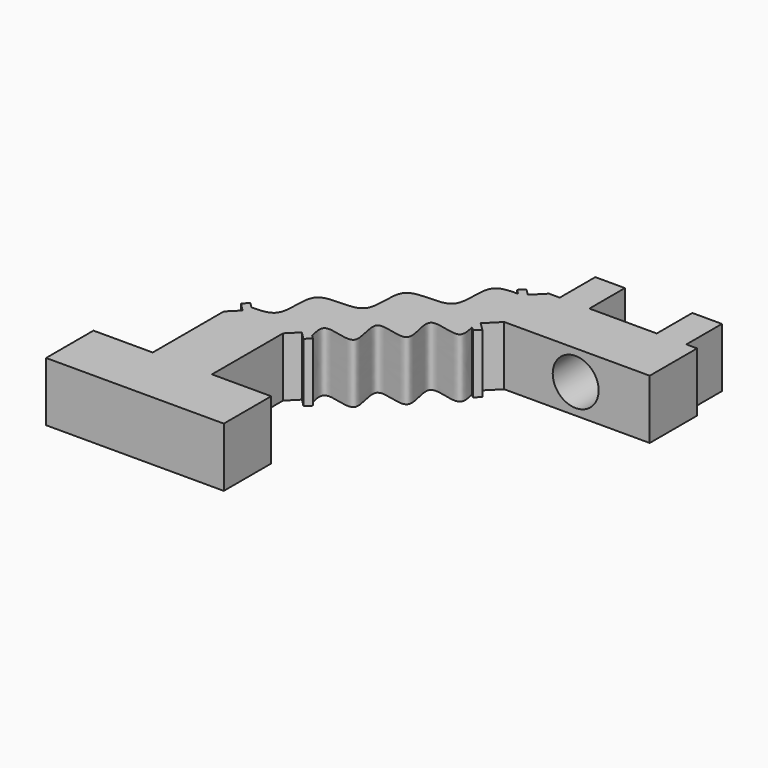
from build123d import *

# Parameters (mm, degrees)
F1_DEPTH = 4
F2_W     = 2
F2_H     = 4
F3_DEPTH = 3
F4_R     = 1.55
F5_DEPTH = 4


# Not quite as in the source:
# - ends of sketch curves that miss each other by under 0.0002 mm in the source are joined


with BuildPart() as f1:
    # F0 (on Top) → F1 (new body)
    with BuildSketch(Plane.XY):
        with BuildLine():
            Line((4, 0), (8, 0))
            Line((8, 0), (12, 0))
            Line((12, 0), (12, 4))
            Line((12, 4), (8, 4))
            Line((8, 4), (8, 10))
            Line((8, 10), (8.7071067812, 10.7071067812))
            Line((8.7071067812, 10.7071067812), (8.1767766953, 11.2374368671))
            Line((8.1767766953, 11.2374368671), (8.5303300859, 11.5909902577))
            Line((8.5303300859, 11.5909902577), (8.7778174593, 11.3435028843))
            add(Edge.make_bspline(
                [(8.7778174593, 11.3435028843), (8.6793135956, 11.7753291065), (8.4823058683, 12.638981551), (9.7777845344, 12.3434699588), (10.6414369797, 12.1464622341), (10.8080981583, 12.3131234115)],
                knots=[0, 0, 0, 0, 0.0833326877, 0.1666653755, 0.2499980632, 0.2499980632, 0.2499980632, 0.2499980632], degree=3))
            add(Edge.make_bspline(
                [(10.8080981583, 12.3131234115), (10.9747593369, 12.4797845889), (10.7777516061, 13.3434370232), (10.4822400343, 14.6389157463), (11.7777186285, 14.343403944), (13.0731975651, 14.047893141), (12.7776849661, 15.3433688663), (12.4821771366, 16.6388585097), (13.7776618368, 16.3433013729), (15.073233045, 16.047933522), (14.8762893212, 16.9116464302), (14.7778174593, 17.3435028843)],
                knots=[0.2499980632, 0.2499980632, 0.2499980632, 0.2499980632, 0.333330751, 0.4166634387, 0.4999961264, 0.5833288142, 0.6666615019, 0.7499941897, 0.8333268774, 0.9166634387, 1, 1, 1, 1], degree=3))
            Line((14.7778174593, 17.3435028843), (14.5303300859, 17.5909902577))
            Line((14.5303300859, 17.5909902577), (14.8838834765, 17.9445436483))
            Line((14.8838834765, 17.9445436483), (15.4142135624, 17.4142135624))
            Line((15.4142135624, 17.4142135624), (16.2980970389, 18.2980970389))
            Line((16.2980970389, 18.2980970389), (26.1212241882, 18.2980970389))
            Line((26.1212241882, 18.2980970389), (26.1212241882, 22.2980970389))
            Line((26.1212241882, 22.2980970389), (16.1212241882, 22.2980970389))
            Line((16.1212241882, 22.2980970389), (15.3256809034, 21.5025539105))
            Line((15.3256809034, 21.5025539105), (15.7675746595, 21.0606601544))
            Line((15.7675746595, 21.0606601544), (15.4140212689, 20.7071067638))
            Line((15.4140212689, 20.7071067638), (15.3257290593, 20.7953989734))
            Line((15.3257290593, 20.7953989734), (15.2726959638, 20.8484320689))
            add(Edge.make_bspline(
                [(5.2727919408, 10.8485280459), (5.8157320976, 10.8611381168), (6.9016124112, 10.8863582587), (6.939442624, 12.5151787291), (6.9772728368, 14.1439991996), (8.6060933073, 14.1818294124), (10.2349137777, 14.2196596252), (10.2727439905, 15.8484800956), (10.3105742033, 17.4773005661), (11.9393946738, 17.5151307789), (13.5682151443, 17.5529609917), (13.6060453571, 19.1817814621), (13.6438755698, 20.8106019326), (14.7297558835, 20.8358220745), (15.2726959638, 20.8484320689)],
                knots=[0, 0, 0, 0, 0.0833333333, 0.1666666667, 0.25, 0.3333333333, 0.4166666667, 0.5, 0.5833333333, 0.6666666667, 0.75, 0.8333333333, 0.9166666667, 1, 1, 1, 1], degree=3))
            Line((5.2727919408, 10.8485280459), (5.6282136765, 10.4931061393))
            Line((5.6282136765, 10.4931061393), (5.2746603207, 10.1395527139))
            Line((5.2746603207, 10.1395527139), (4.7071065842, 10.7071067232))
            Line((4.7071065842, 10.7071067232), (4, 10))
            Line((4, 10), (4, 4))
            Line((4, 4), (0, 4))
            Line((0, 4), (0, 0))
            Line((0, 0), (4, 0))
        make_face()
        Polygon((8.1767766953, 11.2374368671), (8.7071067812, 10.7071067812), (9.2374368671, 10.1767766953), (9.5909902577, 10.5303300859), (9.3435028843, 10.7778174593), (9.0606601718, 11.0606601718), (8.7778174593, 11.3435028843), (8.5303300859, 11.5909902577), align=None)
        Polygon((4.1395527627, 11.2746608175), (4.7071065842, 10.7071067232), (4.8838832621, 10.8838834359), (5.0606599574, 11.0606601312), (4.848527974, 11.2727922166), (4.7954948913, 11.3258253248), (4.4931062383, 11.6282141232), align=None)
        Polygon((4.8838832621, 10.8838834359), (4.7071065842, 10.7071067232), (5.2746603207, 10.1395527139), (5.6282136765, 10.4931061393), (5.2727919408, 10.8485280459), (5.0606599574, 11.0606601312), align=None)
        with BuildLine():
            Line((4.848527974, 11.2727922166), (5.0606599574, 11.0606601312))
            Line((5.0606599574, 11.0606601312), (5.2727919408, 10.8485280459))
            add(Edge.make_bspline(
                [(5.2727919408, 10.8485280459), (5.8157320976, 10.8611381168), (6.9016124112, 10.8863582587), (6.939442624, 12.5151787291), (6.9772728368, 14.1439991996), (8.6060933073, 14.1818294124), (10.2349137777, 14.2196596252), (10.2727439905, 15.8484800956), (10.3105742033, 17.4773005661), (11.9393946738, 17.5151307789), (13.5682151443, 17.5529609917), (13.6060453571, 19.1817814621), (13.6438755698, 20.8106019326), (14.7297558835, 20.8358220745), (15.2726960403, 20.8484321454)],
                knots=[0, 0, 0, 0, 0.0833333333, 0.1666666667, 0.25, 0.3333333333, 0.4166666667, 0.5, 0.5833333333, 0.6666666667, 0.75, 0.8333333333, 0.9166666667, 1, 1, 1, 1], degree=3))
            Line((15.2726960403, 20.8484321454), (14.8484318951, 21.2726961376))
            add(Edge.make_bspline(
                [(4.848527974, 11.2727922166), (5.3914681818, 11.2854023385), (6.4773484955, 11.3106224803), (6.5151787083, 12.9394429508), (6.5530089211, 14.5682634213), (8.1818293915, 14.6060936341), (9.810649862, 14.6439238468), (9.8484800748, 16.2727443173), (9.8863102876, 17.9015647878), (11.5151307581, 17.9393950006), (13.1439512285, 17.9772252134), (13.1817814413, 19.6060456838), (13.2196116541, 21.2348661543), (14.3054919677, 21.2600862962), (14.8484318951, 21.2726961376)],
                knots=[0, 0, 0, 0, 0.0833333333, 0.1666666667, 0.25, 0.3333333333, 0.4166666667, 0.5, 0.5833333333, 0.6666666667, 0.75, 0.8333333333, 0.9166666667, 1, 1, 1, 1], degree=3))
        make_face()
        with BuildLine():
            add(Edge.make_bspline(
                [(8.7778174593, 11.3435028843), (8.6793135956, 11.7753291065), (8.4823058683, 12.638981551), (9.7777845344, 12.3434699588), (10.6414369797, 12.1464622341), (10.8080981583, 12.3131234115)],
                knots=[0, 0, 0, 0, 0.0833326877, 0.1666653755, 0.2499980632, 0.2499980632, 0.2499980632, 0.2499980632], degree=3))
            Line((8.7778174593, 11.3435028843), (9.0606601718, 11.0606601718))
            Line((9.0606601718, 11.0606601718), (9.3435028843, 10.7778174593))
            add(Edge.make_bspline(
                [(9.3435028843, 10.7778174593), (9.2449990206, 11.2096436816), (9.0479912932, 12.0732961261), (10.3434699594, 11.7777845339), (11.6389486273, 11.4822729468), (11.343437031, 12.7777515982), (11.0479254593, 14.0732303213), (12.3434040535, 13.777718519), (13.6388829901, 13.482207716), (13.343370391, 14.7776834413), (13.0478625616, 16.0731730848), (14.3433472618, 15.7776159479), (15.6389184699, 15.4822480971), (15.4419747461, 16.3459610052), (15.3435028843, 16.7778174593)],
                knots=[0, 0, 0, 0, 0.0833326877, 0.1666653755, 0.2499980632, 0.333330751, 0.4166634387, 0.4999961264, 0.5833288142, 0.6666615019, 0.7499941897, 0.8333268774, 0.9166634387, 1, 1, 1, 1], degree=3))
            Line((15.3435028843, 16.7778174593), (14.7778174593, 17.3435028843))
            add(Edge.make_bspline(
                [(10.8080981583, 12.3131234115), (10.9747593369, 12.4797845889), (10.7777516061, 13.3434370232), (10.4822400343, 14.6389157463), (11.7777186285, 14.343403944), (13.0731975651, 14.047893141), (12.7776849661, 15.3433688663), (12.4821771366, 16.6388585097), (13.7776618368, 16.3433013729), (15.073233045, 16.047933522), (14.8762893212, 16.9116464302), (14.7778174593, 17.3435028843)],
                knots=[0.2499980632, 0.2499980632, 0.2499980632, 0.2499980632, 0.333330751, 0.4166634387, 0.4999961264, 0.5833288142, 0.6666615019, 0.7499941897, 0.8333268774, 0.9166634387, 1, 1, 1, 1], degree=3))
        make_face()
        Polygon((14.7778174593, 17.3435028843), (15.3435028843, 16.7778174593), (15.5909902577, 16.5303300859), (15.9445436483, 16.8838834765), (15.4142135624, 17.4142135624), (14.8838834765, 17.9445436483), (14.5303300859, 17.5909902577), align=None)
        Polygon((14.7953989734, 21.3257290593), (14.8484318951, 21.2726961376), (15.2726959638, 20.8484320689), (15.3257290593, 20.7953989734), (15.4140212689, 20.7071067638), (15.7675746595, 21.0606601544), (15.3256809034, 21.5025539105), (14.8837871473, 21.9444476667), (14.5302337567, 21.5908942761), align=None)
    extrude(amount=F1_DEPTH)

    # F2 (on face) → F3 (join)
    with BuildSketch(Plane(origin=(0, 22.2980970389, 0), x_dir=(-1, 0, 0), z_dir=(0, 1, 0))):
        with Locations((-24.3962241882, 2)):
            Rectangle(F2_W, F2_H)
        with Locations((-17.8462241882, 2)):
            Rectangle(F2_W, F2_H)
    extrude(amount=F3_DEPTH)

    # F4 (on face) → F5 (cut)
    with BuildSketch(Plane(origin=(0, 22.2980970389, 0), x_dir=(-1, 0, 0), z_dir=(0, 1, 0))):
        with Locations((-21.1212241882, 2)):
            Circle(F4_R)
    extrude(amount=-F5_DEPTH, mode=Mode.SUBTRACT)


with BuildPart() as f6_1:
    # F6: copy of F1
    add(f1.part)


solid = Compound([f1.part, f6_1.part])
